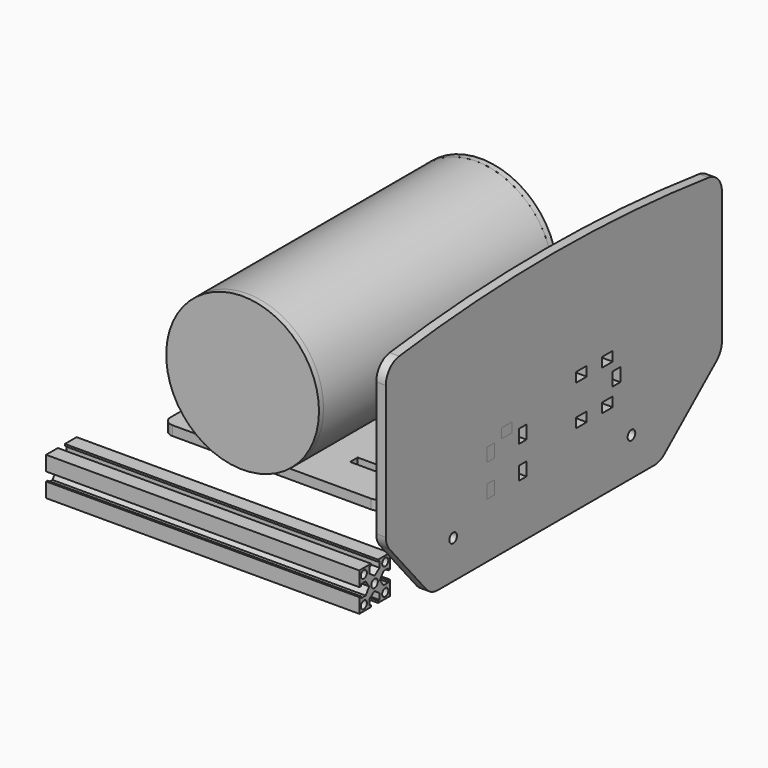
from build123d import *

# Parameters (mm, degrees)
F0_R           = 40
F0_R_2         = 37
F1_DEPTH       = 150
F2_R           = 40
F3_DEPTH       = 3
F4_R           = 32
F4_R_2         = 27
F5_DEPTH       = 5
F6_R           = 40
F7_DEPTH       = 3
F8_R           = 32.7
F9_DEPTH       = 6
F10_R          = 36.5
F11_DEPTH      = 3
F12_R          = 36.5
F12_R_2        = 1.5
F12_R_3        = 1.05
F12_W          = 9
F12_H          = 9
F13_DEPTH      = 3
F14_R          = 2
F14_R_2        = 2.15
F15_DEPTH      = 82
F15_DEPTH_BACK = 82
F16_R          = 2.5
F17_DEPTH      = 5
F18_R          = 2
F18_W          = 15
F18_H          = 5
F18_W_2        = 5
F18_H_2        = 15
F19_DEPTH      = 5
F21_DEPTH      = 5
F22_R          = 5
F23_W          = 15
F23_H          = 5
F24_DEPTH      = 5
F25_W          = 5
F25_H          = 7
F25_W_2        = 7
F25_H_2        = 5
F26_DEPTH      = 25
F27_R          = 1
F27_R_2        = 5.5
F27_W          = 5
F27_H          = 7
F28_DEPTH      = 5
F29_W          = 5
F29_H          = 7
F29_W_2        = 8
F29_H_2        = 5
F30_DEPTH      = 5


# Not quite as in the source:
# - a feature names something its author has since deleted; it is built from what else it names


with BuildPart() as f1:
    # F0 (on Front) → F1 (new body)
    with BuildSketch(Plane.XZ):
        Circle(F0_R)
        Circle(F0_R_2, mode=Mode.SUBTRACT)
    extrude(amount=F1_DEPTH)


with BuildPart() as f3:
    # F2 (on face) → F3 (new body)
    with BuildSketch(Plane.XZ.offset(150)):
        Circle(F2_R)
    extrude(amount=F3_DEPTH)


with BuildPart() as f5:
    # F4 (on face) → F5 (new body)
    with BuildSketch(Plane(origin=(0, -150, 0), x_dir=(-1, 0, 0), z_dir=(0, 1, 0))):
        Circle(F4_R)
        Circle(F4_R_2, mode=Mode.SUBTRACT)
    extrude(amount=F5_DEPTH)


with BuildPart() as f7:
    # F6 (on face) → F7 (new body)
    with BuildSketch(Plane(origin=(0, 0, 0), x_dir=(-1, 0, 0), z_dir=(0, 1, 0))):
        Circle(F6_R)
    extrude(amount=F7_DEPTH)


with BuildPart() as f9:
    # F8 (on face) → F9 (new body)
    with BuildSketch(Plane.XZ):
        Circle(F8_R)
    extrude(amount=F9_DEPTH)


with BuildPart() as f11:
    # F10 (on face) → F11 (new body)
    with BuildSketch(Plane.XZ.offset(6)):
        Circle(F10_R)
    extrude(amount=F11_DEPTH)


with BuildPart() as f13:
    # F12 (on face) → F13 (new body)
    with BuildSketch(Plane(origin=(0, -145, 0), x_dir=(-1, 0, 0), z_dir=(0, 1, 0))):
        Circle(F12_R)
        with Locations((-14, -30)):
            Circle(F12_R_2, mode=Mode.SUBTRACT)
        with Locations((-12.4, -10.5)):
            Circle(F12_R_3, mode=Mode.SUBTRACT)
        with Locations((0.1, -10.5)):
            Circle(F12_R_3, mode=Mode.SUBTRACT)
        with Locations((-12.4, 10.5)):
            Circle(F12_R_3, mode=Mode.SUBTRACT)
        with Locations((-14, 30)):
            Circle(F12_R_2, mode=Mode.SUBTRACT)
        Rectangle(F12_W, F12_H, mode=Mode.SUBTRACT)
        with Locations((0.1, 10.5)):
            Circle(F12_R_3, mode=Mode.SUBTRACT)
        with Locations((28, 0)):
            Circle(F12_R_2, mode=Mode.SUBTRACT)
    extrude(amount=F13_DEPTH)


with BuildPart() as f15:
    # F14 (on Right) → F15 (new body, two sides)
    with BuildSketch(Plane.YZ) as f15_sk:
        Polygon((-159.1363453865, -56.8636933386), (-159.1363453865, -49.1636933386), (-166.8363453865, -49.1636933386), (-166.8363453865, -50.1636933386), (-165.8363453865, -50.1636933386), (-165.8363453865, -53.3625178193), (-169.1363453865, -55.6636933386), (-172.4363453865, -53.3625178193), (-172.4363453865, -50.1636933386), (-171.4363453865, -50.1636933386), (-171.4363453865, -49.1636933386), (-179.1363453865, -49.1636933386), (-179.1363453865, -56.8636933386), (-178.1363453865, -56.8636933386), (-178.1363453865, -55.8636933386), (-174.9375209058, -55.8636933386), (-172.6363453865, -59.1636933386), (-174.9375209058, -62.4636933386), (-178.1363453865, -62.4636933386), (-178.1363453865, -61.4636933386), (-179.1363453865, -61.4636933386), (-179.1363453865, -69.1636933386), (-171.4363453865, -69.1636933386), (-171.4363453865, -68.1636933386), (-172.4363453865, -68.1636933386), (-172.4363453865, -64.964868858), (-169.1363453865, -62.6636933386), (-165.8363453865, -64.964868858), (-165.8363453865, -68.1636933386), (-166.8363453865, -68.1636933386), (-166.8363453865, -69.1636933386), (-159.1363453865, -69.1636933386), (-159.1363453865, -61.4636933386), (-160.1363453865, -61.4636933386), (-160.1363453865, -62.4636933386), (-163.3351698672, -62.4636933386), (-165.6363453865, -59.1636933386), (-163.3351698672, -55.8636933386), (-160.1363453865, -55.8636933386), (-160.1363453865, -56.8636933386), align=None)
        with Locations((-176.1363453865, -66.1636933386)):
            Circle(F14_R, mode=Mode.SUBTRACT)
        with Locations((-162.1363453865, -66.1636933386)):
            Circle(F14_R, mode=Mode.SUBTRACT)
        with Locations((-176.1363453865, -52.1636933386)):
            Circle(F14_R, mode=Mode.SUBTRACT)
        with Locations((-169.1363453865, -59.1636933386)):
            Circle(F14_R_2, mode=Mode.SUBTRACT)
        with Locations((-162.1363453865, -52.1636933386)):
            Circle(F14_R, mode=Mode.SUBTRACT)
    extrude(amount=F15_DEPTH)
    extrude(f15_sk.sketch, amount=-F15_DEPTH_BACK)


with BuildPart() as f17:
    # F16 (on face) → F17 (new body)
    with BuildSketch(Plane.YZ.offset(82)):
        with BuildLine():
            Line((-165.6096495469, -43.2440153403), (-141.5291008976, -71.4879298526))
            ThreePointArc((-141.5291008976, -71.4879298526), (-138.1099585678, -74.0796282558), (-133.9194513506, -75))
            Line((-133.9194513506, -75), (7.7809598532, -75))
            ThreePointArc((7.7809598532, -75), (11.2380904936, -74.3834027802), (14.2688897058, -72.6096495469))
            Line((14.2688897058, -72.6096495469), (48.4879298526, -43.4347538139))
            ThreePointArc((48.4879298526, -43.4347538139), (51.0796282558, -40.0156114841), (52, -35.8251042669))
            Line((52, -35.8251042669), (52, 33.2439145123))
            ThreePointArc((52, 33.2439145123), (49.5052724084, 39.8523096334), (43.2658227848, 43.1634756255))
            ThreePointArc((43.2658227848, 43.1634756255), (-58, 49.5985865737), (-159.2658227848, 43.1634756255))
            ThreePointArc((-159.2658227848, 43.1634756254), (-165.5052724084, 39.8523096334), (-168, 33.2439145123))
            Line((-168, 33.2439145123), (-168, -36.7560854877))
            ThreePointArc((-168, -36.7560854877), (-167.3834027802, -40.2132161282), (-165.6096495469, -43.2440153403))
        make_face()
        with Locations((-123.9194513506, -55)):
            Circle(F16_R, mode=Mode.SUBTRACT)
        with Locations((-7.2190401468, -55)):
            Circle(F16_R, mode=Mode.SUBTRACT)
    extrude(amount=F17_DEPTH)

    # F25 (on face) → F26 (cut)
    with BuildSketch(Plane.YZ.offset(87)):
        with Locations((-99.4194513506, -25.6636933386)):
            Rectangle(F25_W, F25_H)
        with Locations((-99.4194513506, -42.6636933386)):
            Rectangle(F25_W, F25_H)
        with Locations((-78.4194513506, -42.6636933386)):
            Rectangle(F25_W, F25_H)
        with Locations((-78.4194513506, -25.6636933386)):
            Rectangle(F25_W, F25_H)
        with Locations((-88.9194513506, -19.6636933386)):
            Rectangle(F25_W_2, F25_H_2)
        with Locations((-17, -24.1636933386)):
            Rectangle(F25_W, F25_H)
        with Locations((-23, -13.6636933386)):
            Rectangle(F25_W_2, F25_H_2)
        with Locations((-40, -13.6636933386)):
            Rectangle(F25_W_2, F25_H_2)
        with Locations((-23, -34.6636933386)):
            Rectangle(F25_W_2, F25_H_2)
        with Locations((-40, -34.6636933386)):
            Rectangle(F25_W_2, F25_H_2)
    extrude(amount=-F26_DEPTH, mode=Mode.SUBTRACT)


with BuildPart() as f19:
    # F18 (on face) → F19 (new body)
    with BuildSketch(Plane.XY.offset(-49.1636933386)):
        Polygon((57, 2.7809598532), (-57, 2.7809598532), (-57, -17.2190401468), (-46, -29.5692457487), (-46, -101.5692457487), (-57, -113.9194513506), (-57, -133.9194513506), (57, -133.9194513506), (57, -113.9194513506), (46, -101.5692457487), (46, -29.5692457487), (57, -17.2190401468), align=None)
        with Locations((-50, -123.9194513506)):
            Circle(F18_R, mode=Mode.SUBTRACT)
        with Locations((-32.5, -111.4194513506)):
            Rectangle(F18_W, F18_H, mode=Mode.SUBTRACT)
        with Locations((-32.5, -93.9194513506)):
            Rectangle(F18_W_2, F18_H_2, mode=Mode.SUBTRACT)
        with Locations((32.5, -111.4194513506)):
            Rectangle(F18_W, F18_H, mode=Mode.SUBTRACT)
        with Locations((32.5, -93.9194513506)):
            Rectangle(F18_W_2, F18_H_2, mode=Mode.SUBTRACT)
        with Locations((50, -123.9194513506)):
            Circle(F18_R, mode=Mode.SUBTRACT)
        with Locations((-50, -7.2190401468)):
            Circle(F18_R, mode=Mode.SUBTRACT)
        with Locations((-32.5, -37.2190401468)):
            Rectangle(F18_W_2, F18_H_2, mode=Mode.SUBTRACT)
        with Locations((-32.5, -19.7190401468)):
            Rectangle(F18_W, F18_H, mode=Mode.SUBTRACT)
        with Locations((32.5, -37.2190401468)):
            Rectangle(F18_W_2, F18_H_2, mode=Mode.SUBTRACT)
        with Locations((32.5, -19.7190401468)):
            Rectangle(F18_W, F18_H, mode=Mode.SUBTRACT)
        with Locations((50, -7.2190401468)):
            Circle(F18_R, mode=Mode.SUBTRACT)
    extrude(amount=F19_DEPTH)

    # F22
    f22_edges = [f19.edges().sort_by_distance(p)[0] for p in [
        (-57, 2.78096, -46.663693),
        (57, 2.78096, -46.663693),
        (-57, -133.919451, -46.663693),
        (57, -133.919451, -46.663693),
    ]]
    fillet(f22_edges, radius=F22_R)


with BuildPart() as f21:
    # F20 (on face) → F21 (new body)
    with BuildSketch(Plane(origin=(0, -22.2190401468, 0), x_dir=(-1, 0, 0), z_dir=(0, 1, 0))):
        with BuildLine():
            ThreePointArc((-31.1111111111, -27.3052677808), (-36.6666666667, -25.7339193782), (-40, -30.4479645861))
            Line((-40, -30.4479645861), (-40, -44.1636933386))
            Line((-40, -44.1636933386), (-25, -44.1636933386))
            Line((-25, -44.1636933386), (25, -44.1636933386))
            Line((25, -44.1636933386), (25, -56.1636933386))
            ThreePointArc((25, -56.1636933386), (25.8786796564, -58.2850136822), (28, -59.1636933386))
            Line((28, -59.1636933386), (30, -59.1636933386))
            Line((30, -59.1636933386), (30, -49.1636933386))
            Line((30, -49.1636933386), (35, -49.1636933386))
            Line((35, -49.1636933386), (35, -59.1636933386))
            Line((35, -59.1636933386), (37, -59.1636933386))
            ThreePointArc((37, -59.1636933386), (39.1213203436, -58.2850136822), (40, -56.1636933386))
            Line((40, -56.1636933386), (40, -30.4479645861))
            ThreePointArc((40, -30.4479645861), (36.6666666667, -25.7339193782), (31.1111111111, -27.3052677808))
            ThreePointArc((31.1111111111, -27.3052677808), (0, -42.1636933386), (-31.1111111111, -27.3052677808))
        make_face()
        Polygon((-25, -44.1636933386), (-40, -44.1636933386), (-40, -49.1636933386), (-35, -49.1636933386), (-30, -49.1636933386), (-25, -49.1636933386), align=None)
        with BuildLine():
            Line((-35, -49.1636933386), (-40, -49.1636933386))
            Line((-40, -49.1636933386), (-40, -56.1636933386))
            ThreePointArc((-40, -56.1636933386), (-39.1213203436, -58.2850136822), (-37, -59.1636933386))
            Line((-37, -59.1636933386), (-35, -59.1636933386))
            Line((-35, -59.1636933386), (-35, -49.1636933386))
        make_face()
        with BuildLine():
            Line((-25, -56.1636933386), (-25, -49.1636933386))
            Line((-25, -49.1636933386), (-30, -49.1636933386))
            Line((-30, -49.1636933386), (-30, -59.1636933386))
            Line((-30, -59.1636933386), (-28, -59.1636933386))
            ThreePointArc((-28, -59.1636933386), (-25.8786796564, -58.2850136822), (-25, -56.1636933386))
        make_face()
    extrude(amount=F21_DEPTH)


with BuildPart() as f24:
    # F23 (on face) → F24 (new body)
    with BuildSketch(Plane(origin=(35, 0, 0), x_dir=(0, -1, 0), z_dir=(-1, 0, 0))):
        with BuildLine():
            Line((29.7190401468, -49.1636933386), (17.2190401468, -49.1636933386))
            Line((17.2190401468, -49.1636933386), (17.2190401468, -59.1636933386))
            Line((17.2190401468, -59.1636933386), (22.2190401468, -59.1636933386))
            ThreePointArc((22.2190401468, -59.1636933386), (23.8630300199, -59.027632577), (25.4622833901, -58.6231527981))
            ThreePointArc((25.4622833901, -58.6231527981), (38.6561236941, -55.2861946225), (52.2190401468, -54.1636933386))
            ThreePointArc((52.2190401468, -54.1636933386), (55.7545740528, -52.6992272446), (57.2190401468, -49.1636933386))
            Line((57.2190401468, -49.1636933386), (44.7190401468, -49.1636933386))
            Line((44.7190401468, -49.1636933386), (29.7190401468, -49.1636933386))
        make_face()
        with Locations((37.2190401468, -46.6636933386)):
            Rectangle(F23_W, F23_H)
    extrude(amount=F24_DEPTH)


with BuildPart() as f28:
    # F27 (on face) → F28 (new body)
    with BuildSketch(Plane.XY.offset(-22.1636933386)):
        with BuildLine():
            Line((82, -96.9194513506), (82, -92.4194513506))
            Line((82, -92.4194513506), (82, -85.4194513506))
            Line((82, -85.4194513506), (82, -80.9194513506))
            Line((82, -80.9194513506), (74, -80.9194513506))
            Line((74, -80.9194513506), (74, -75.9194513506))
            Line((74, -75.9194513506), (57.5, -75.9194513506))
            ThreePointArc((57.5, -75.9194513506), (66.6923881554, -79.7270631952), (70.5, -88.9194513506))
            ThreePointArc((70.5, -88.9194513506), (66.6923881554, -98.111839506), (57.5, -101.9194513506))
            Line((57.5, -101.9194513506), (74, -101.9194513506))
            Line((74, -101.9194513506), (74, -96.9194513506))
            Line((74, -96.9194513506), (82, -96.9194513506))
        make_face()
        with BuildLine():
            ThreePointArc((57.5, -75.9194513506), (44.5, -88.9194513506), (57.5, -101.9194513506))
            ThreePointArc((57.5, -101.9194513506), (66.6923881554, -98.111839506), (70.5, -88.9194513506))
            ThreePointArc((70.5, -88.9194513506), (66.6923881554, -79.7270631952), (57.5, -75.9194513506))
        make_face()
        with Locations((62.5, -97.5797053885)):
            Circle(F27_R, mode=Mode.SUBTRACT)
        with Locations((47.5, -88.9194513506)):
            Circle(F27_R, mode=Mode.SUBTRACT)
        with Locations((57.5, -88.9194513506)):
            Circle(F27_R_2, mode=Mode.SUBTRACT)
        with Locations((62.5, -80.2591973128)):
            Circle(F27_R, mode=Mode.SUBTRACT)
        with Locations((84.5, -88.9194513506)):
            Rectangle(F27_W, F27_H)
    extrude(amount=F28_DEPTH)


with BuildPart() as f30:
    # F29 (on face) → F30 (new body)
    with BuildSketch(Plane.XZ.offset(96.9194513506)):
        with Locations((84.5, -25.6636933386)):
            Rectangle(F29_W, F29_H)
        with BuildLine():
            Line((82, -29.1636933386), (82, -22.1636933386))
            Line((82, -22.1636933386), (74, -22.1636933386))
            Line((74, -22.1636933386), (67.5, -22.1636933386))
            Line((67.5, -22.1636933386), (67.5, -27.8625702385))
            ThreePointArc((67.5, -27.8625702385), (67.5835862635, -29.1528177368), (67.8329477214, -30.4214958416))
            Line((67.8329477214, -30.4214958416), (70.0303038361, -38.7226189418))
            ThreePointArc((70.0303038361, -38.7226189418), (73.5977354721, -44.0879994922), (79.6973561147, -46.1636933386))
            Line((79.6973561147, -46.1636933386), (82, -46.1636933386))
            Line((82, -46.1636933386), (82, -39.1636933386))
            Line((82, -39.1636933386), (82, -29.1636933386))
        make_face()
        with Locations((78, -19.6636933386)):
            Rectangle(F29_W_2, F29_H_2)
        with Locations((84.5, -42.6636933386)):
            Rectangle(F29_W, F29_H)
    extrude(amount=F30_DEPTH)


solid = Compound([f1.part, f3.part, f5.part, f7.part, f9.part, f11.part, f13.part, f15.part, f17.part, f19.part, f21.part, f24.part, f28.part, f30.part])
